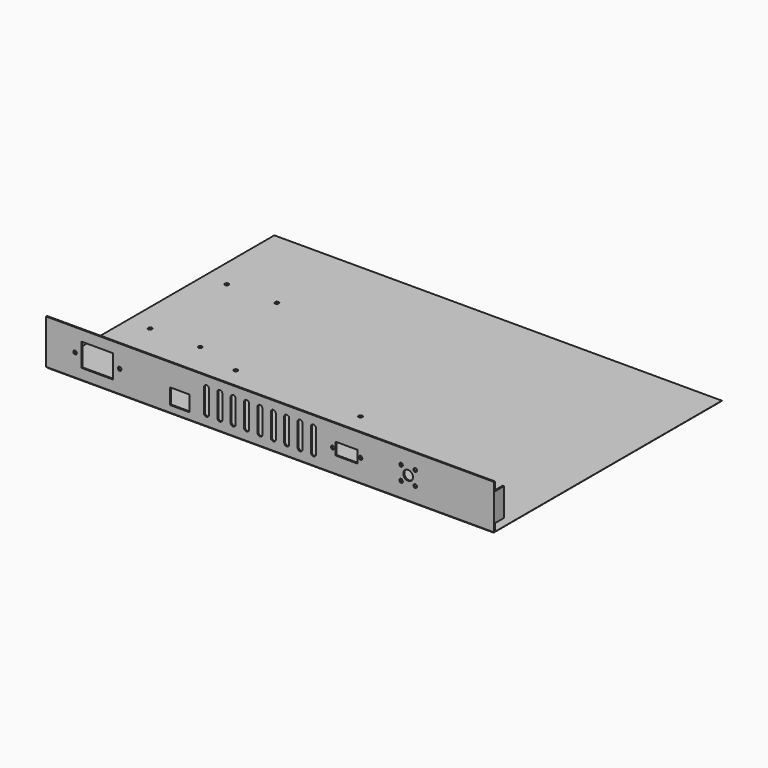
from build123d import *

# Parameters (mm, degrees)
F0_W         = 402
F0_H         = 41
F0_W_2       = 17.5
F0_H_2       = 14
F0_R         = 1.6
F0_W_3       = 28
F0_H_3       = 20.8
F0_W_4       = 19.6
F0_H_4       = 10.9
F0_R_2       = 4.35
F1_DEPTH     = 1.1
F2_W         = 1.1
F2_H         = 25.2
F3_DEPTH     = 10.1
F4_W         = 402
F4_H         = 1.1
F5_DEPTH     = 255
F7_D         = 3.2
F9_D         = 3.2
F10_T1_DEPTH = 408.1720391711
F10_T3_DEPTH = 262.2720391711


# Not quite as in the source:
# - a fillet or chamfer that OpenCascade refuses, or shapes differently, is made with other operations: its cross-section is extruded or revolved along the edge and cut away or added


with BuildPart() as f1:
    # F0 (on Front) → F1 (new body)
    with BuildSketch(Plane.XZ):
        with Locations((201, -20.5)):
            Rectangle(F0_W, F0_H)
        with Locations((120, -26.8)):
            Rectangle(F0_W_2, F0_H_2, mode=Mode.SUBTRACT)
        with Locations((318.65, -26.25)):
            Circle(F0_R, mode=Mode.SUBTRACT)
        with Locations((331.35, -26.25)):
            Circle(F0_R, mode=Mode.SUBTRACT)
        with Locations((26, -19.9)):
            Circle(F0_R, mode=Mode.SUBTRACT)
        with Locations((46, -19.9)):
            Rectangle(F0_W_3, F0_H_3, mode=Mode.SUBTRACT)
        with Locations((66, -19.9)):
            Circle(F0_R, mode=Mode.SUBTRACT)
        with BuildLine():
            ThreePointArc((141.75, -9.65), (144, -7.4), (146.25, -9.65))
            Line((146.25, -9.65), (146.25, -30.15))
            ThreePointArc((146.25, -30.15), (144, -32.4), (141.75, -30.15))
            Line((141.75, -30.15), (141.75, -9.65))
        make_face(mode=Mode.SUBTRACT)
        with BuildLine():
            ThreePointArc((153.75, -9.65), (156, -7.4), (158.25, -9.65))
            Line((158.25, -9.65), (158.25, -30.15))
            ThreePointArc((158.25, -30.15), (156, -32.4), (153.75, -30.15))
            Line((153.75, -30.15), (153.75, -9.65))
        make_face(mode=Mode.SUBTRACT)
        with BuildLine():
            ThreePointArc((165.75, -9.65), (168, -7.4), (170.25, -9.65))
            Line((170.25, -9.65), (170.25, -30.15))
            ThreePointArc((170.25, -30.15), (168, -32.4), (165.75, -30.15))
            Line((165.75, -30.15), (165.75, -9.65))
        make_face(mode=Mode.SUBTRACT)
        with BuildLine():
            ThreePointArc((177.75, -9.65), (180, -7.4), (182.25, -9.65))
            Line((182.25, -9.65), (182.25, -30.15))
            ThreePointArc((182.25, -30.15), (180, -32.4), (177.75, -30.15))
            Line((177.75, -30.15), (177.75, -9.65))
        make_face(mode=Mode.SUBTRACT)
        with BuildLine():
            ThreePointArc((189.75, -9.65), (192, -7.4), (194.25, -9.65))
            Line((194.25, -9.65), (194.25, -30.15))
            ThreePointArc((194.25, -30.15), (192, -32.4), (189.75, -30.15))
            Line((189.75, -30.15), (189.75, -9.65))
        make_face(mode=Mode.SUBTRACT)
        with BuildLine():
            ThreePointArc((201.75, -9.65), (204, -7.4), (206.25, -9.65))
            Line((206.25, -9.65), (206.25, -30.15))
            ThreePointArc((206.25, -30.15), (204, -32.4), (201.75, -30.15))
            Line((201.75, -30.15), (201.75, -9.65))
        make_face(mode=Mode.SUBTRACT)
        with BuildLine():
            ThreePointArc((213.75, -9.65), (216, -7.4), (218.25, -9.65))
            Line((218.25, -9.65), (218.25, -30.15))
            ThreePointArc((218.25, -30.15), (216, -32.4), (213.75, -30.15))
            Line((213.75, -30.15), (213.75, -9.65))
        make_face(mode=Mode.SUBTRACT)
        with BuildLine():
            ThreePointArc((225.75, -9.65), (228, -7.4), (230.25, -9.65))
            Line((230.25, -9.65), (230.25, -30.15))
            ThreePointArc((230.25, -30.15), (228, -32.4), (225.75, -30.15))
            Line((225.75, -30.15), (225.75, -9.65))
        make_face(mode=Mode.SUBTRACT)
        with BuildLine():
            ThreePointArc((237.75, -9.65), (240, -7.4), (242.25, -9.65))
            Line((242.25, -9.65), (242.25, -30.15))
            ThreePointArc((242.25, -30.15), (240, -32.4), (237.75, -30.15))
            Line((237.75, -30.15), (237.75, -9.65))
        make_face(mode=Mode.SUBTRACT)
        with Locations((257.3, -19.9)):
            Circle(F0_R, mode=Mode.SUBTRACT)
        with Locations((269.8, -19.9)):
            Rectangle(F0_W_4, F0_H_4, mode=Mode.SUBTRACT)
        with Locations((282.3, -19.9)):
            Circle(F0_R, mode=Mode.SUBTRACT)
        with Locations((325, -19.9)):
            Circle(F0_R_2, mode=Mode.SUBTRACT)
        with Locations((318.65, -13.55)):
            Circle(F0_R, mode=Mode.SUBTRACT)
        with Locations((331.35, -13.55)):
            Circle(F0_R, mode=Mode.SUBTRACT)
    extrude(amount=F1_DEPTH)

    # F2 (on face) → F3 (join)
    with BuildSketch(Plane(origin=(0, 0, 0), x_dir=(-1, 0, 0), z_dir=(0, 1, 0))):
        with Locations((-401.45, -20.5)):
            Rectangle(F2_W, F2_H)
        with Locations((-0.55, -20.5)):
            Rectangle(F2_W, F2_H)
    extrude(amount=F3_DEPTH)

    # F4 (on face) → F5 (join)
    with BuildSketch(Plane(origin=(0, 0, 0), x_dir=(-1, 0, 0), z_dir=(0, 1, 0))):
        with Locations((-201, -40.45)):
            Rectangle(F4_W, F4_H)
    extrude(amount=F5_DEPTH)

    # F7 (through all)
    with Locations(Plane.XY.offset(-39.9)):
        with Locations((20.5, 90), (65.5, 90), (65.5, 176), (20.5, 176)):
            Hole(F7_D / 2)

    # F9 (through all)
    with Locations(Plane.XY.offset(-39.9)):
        with Locations((106.95, 6), (106.95, 78), (218.95, 6), (218.95, 78)):
            Hole(F9_D / 2)

    # F10: chamfer of 1.2 on 12 edges, made by hand

    # F10_s2 → F10_t1 (cut)
    with BuildSketch(Plane.YZ.offset(-3.0860195856)):
        Polygon((-1.1, -39.8), (0.1, -41), (-1.1, -41), align=None)
        Polygon((253.8, -41), (255, -39.8), (255, -41), align=None)
    extrude(amount=F10_T1_DEPTH, mode=Mode.SUBTRACT)

    # F10_s4 → F10_t3 (cut)
    with BuildSketch(Plane.XZ.offset(-258.0860195856)):
        Polygon((0, -39.8), (1.2, -41), (0, -41), align=None)
        Polygon((402, -39.8), (400.8, -41), (402, -41), align=None)
    extrude(amount=F10_T3_DEPTH, mode=Mode.SUBTRACT)

    # F10_s5 → F10_t6 (revolve, cut)
    with BuildSketch(Plane.XZ.offset(-6)):
        Polygon((109.75, -41), (108.55, -39.8), (108.55, -41), align=None)
    revolve(axis=Axis((106.95, 6, -41), (0, 0, 1)), mode=Mode.SUBTRACT)

    # F10_s7 → F10_t8 (revolve, cut)
    with BuildSketch(Plane.XZ.offset(-90)):
        Polygon((23.3, -41), (22.1, -39.8), (22.1, -41), align=None)
    revolve(axis=Axis((20.5, 90, -41), (0, 0, 1)), mode=Mode.SUBTRACT)

    # F10_s9 → F10_t10 (revolve, cut)
    with BuildSketch(Plane.XZ.offset(-90)):
        Polygon((68.3, -41), (67.1, -39.8), (67.1, -41), align=None)
    revolve(axis=Axis((65.5, 90, -41), (0, 0, 1)), mode=Mode.SUBTRACT)

    # F10_s11 → F10_t12 (revolve, cut)
    with BuildSketch(Plane.XZ.offset(-78)):
        Polygon((109.75, -41), (108.55, -39.8), (108.55, -41), align=None)
    revolve(axis=Axis((106.95, 78, -41), (0, 0, 1)), mode=Mode.SUBTRACT)

    # F10_s13 → F10_t14 (revolve, cut)
    with BuildSketch(Plane.XZ.offset(-6)):
        Polygon((221.75, -41), (220.55, -39.8), (220.55, -41), align=None)
    revolve(axis=Axis((218.95, 6, -41), (0, 0, 1)), mode=Mode.SUBTRACT)

    # F10_s15 → F10_t16 (revolve, cut)
    with BuildSketch(Plane.XZ.offset(-78)):
        Polygon((221.75, -41), (220.55, -39.8), (220.55, -41), align=None)
    revolve(axis=Axis((218.95, 78, -41), (0, 0, 1)), mode=Mode.SUBTRACT)

    # F10_s17 → F10_t18 (revolve, cut)
    with BuildSketch(Plane.XZ.offset(-176)):
        Polygon((23.3, -41), (22.1, -39.8), (22.1, -41), align=None)
    revolve(axis=Axis((20.5, 176, -41), (0, 0, 1)), mode=Mode.SUBTRACT)

    # F10_s19 → F10_t20 (revolve, cut)
    with BuildSketch(Plane.XZ.offset(-176)):
        Polygon((68.3, -41), (67.1, -39.8), (67.1, -41), align=None)
    revolve(axis=Axis((65.5, 176, -41), (0, 0, 1)), mode=Mode.SUBTRACT)


solid = f1.part
